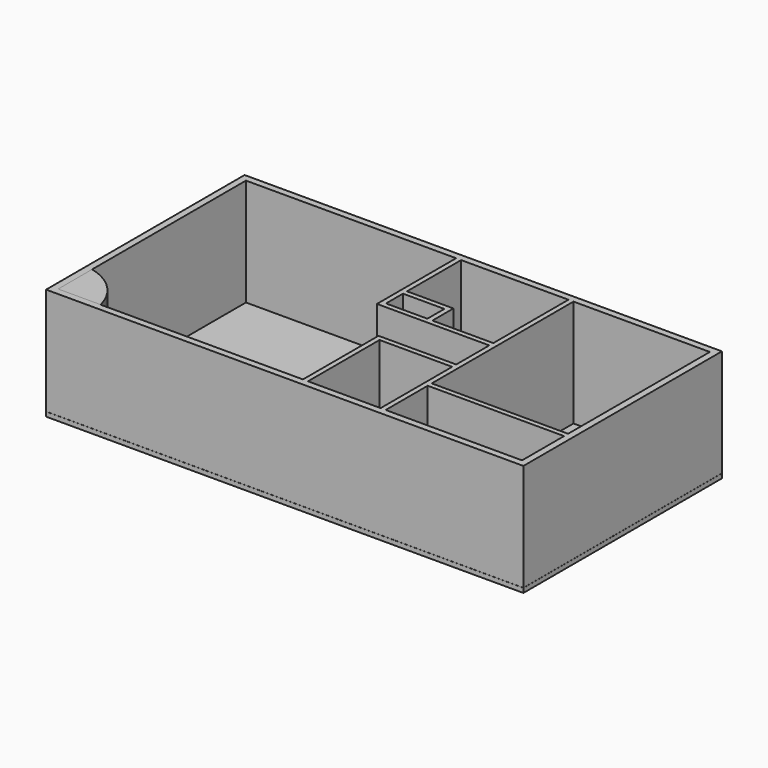
from build123d import *

# Parameters (mm, degrees)
F1_W     = 10845.8
F1_H     = 5638.8
F1_W_2   = 1651
F1_H_2   = 2032
F1_W_3   = 3098.8
F1_H_3   = 1193.8
F1_W_4   = 939.8
F1_H_4   = 482.6
F1_H_5   = 4025.9
F3_DEPTH = 2438.4
F4_W     = 10845.8
F4_H     = 5638.8
F5_DEPTH = 101.6


# Not quite as in the source:
# - a length typed as a fraction of an inch, garbled in the dataset ("3 / 203.2 mm" for 3/8 in), is restored


with BuildPart() as f3:
    # F1 (on Top) → F3 (new body)
    with BuildSketch(Plane.XY):
        with Locations((5422.9, 2819.4)):
            Rectangle(F1_W, F1_H)
        Polygon((4927.6, 5486.4), (4927.6, 3238.5), (5041.9, 3238.5), (7480.3, 3238.5), (7480.3, 2298.7), (5829.3, 2298.7), (5715, 2298.7), (5715, 152.4), (152.4, 152.4), (152.4, 5486.4), align=None, mode=Mode.SUBTRACT)
        with Locations((6654.8, 1168.4)):
            Rectangle(F1_W_2, F1_H_2, mode=Mode.SUBTRACT)
        with Locations((9144, 749.3)):
            Rectangle(F1_W_3, F1_H_3, mode=Mode.SUBTRACT)
        with Locations((5511.8, 3594.1)):
            Rectangle(F1_W_4, F1_H_4, mode=Mode.SUBTRACT)
        with Locations((9144, 3473.45)):
            Rectangle(F1_W_3, F1_H_5, mode=Mode.SUBTRACT)
        Polygon((6096, 3949.7), (5041.9, 3949.7), (5041.9, 5486.4), (7480.3, 5486.4), (7480.3, 3352.8), (6096, 3352.8), (6096, 3835.4), align=None, mode=Mode.SUBTRACT)
    extrude(amount=F3_DEPTH)


with BuildPart() as f3b:
    # F2 (on Top) → F3, piece 2 (new body)
    with BuildSketch(Plane.XY):
        with BuildLine():
            Line((152.4, 152.4), (1117.6, 152.4))
            ThreePointArc((1117.6, 152.4), (769.3507636654, 769.3507636654), (152.4, 1117.6))
            Line((152.4, 1117.6), (152.4, 152.4))
        make_face()
    extrude(amount=F3_DEPTH)


with BuildPart() as f5:
    # F4 (on offset) → F5 (new body)
    with BuildSketch(Plane.XY.offset(-1.5875)):
        with Locations((5422.9, 2819.4)):
            Rectangle(F4_W, F4_H)
    extrude(amount=-F5_DEPTH)


solid = Compound([f3.part, f3b.part, f5.part])
